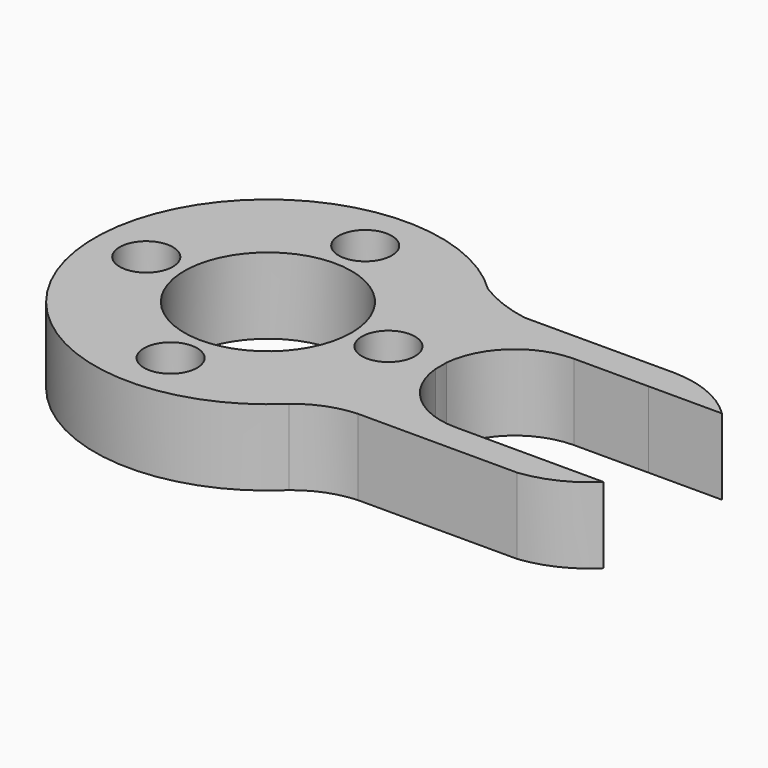
from build123d import *

# Parameters (mm, degrees)
F0_R     = 1.75
F0_R_2   = 5.5
F1_DEPTH = 5


# Not quite as in the source:
# - ends of sketch curves that miss each other by under 0.0002 mm in the source are joined


with BuildPart() as f1:
    # F0 (on Top) → F1 (new body)
    with BuildSketch(Plane.XY):
        with BuildLine():
            ThreePointArc((11.3834703749, 6.8633075193), (9.5916723545, 7.355768815), (7.9272258947, 8.1820110654))
            ThreePointArc((7.9272258947, 8.1820110654), (-11.3923753212, 0), (7.9272258947, -8.1820110654))
            ThreePointArc((7.9272258947, -8.1820110654), (9.5459951376, -7.2276126539), (11.3834703749, -6.8339440851))
            Line((11.3834703749, -6.8339440851), (21.8628461179, -6.8339440851))
            ThreePointArc((21.8628461179, -6.8339440851), (24.0780549828, -6.2025675349), (25.9603803998, -4.874923875))
            Line((25.9603803998, -4.874923875), (21.1398675793, -4.874923875))
            ThreePointArc((21.1398675793, -4.874923875), (21.1127528894, -4.8749999983), (21.0856381954, -4.8749253089))
            ThreePointArc((21.0856381954, -4.8749253089), (21.0855085866, -4.8749245897), (21.0853803998, -4.874923875))
            Line((21.0853803998, -4.874923875), (16.2648675793, -4.874923875))
            ThreePointArc((16.2648675793, -4.874923875), (12.9636398268, -3.6120150473), (11.3834703749, -0.4503528446))
            ThreePointArc((11.3834703749, -0.4503528446), (11.3923753212, 0), (11.3834703749, 0.4503528446))
            ThreePointArc((11.3834703749, 0.4503528446), (12.9535739288, 3.6028655537), (16.2376621588, 4.8749999999))
            Line((16.2376621588, 4.8749999999), (21.1319533126, 4.8749616796))
            Line((21.1319533126, 4.8749616796), (25.9603803998, 4.874923875))
            ThreePointArc((25.9603803998, 4.874923875), (23.8013578283, 6.3274272295), (21.2571545841, 6.8734806254))
            Line((21.2571545841, 6.8734806254), (20.9539298759, 6.8731682053))
            Line((20.9539298759, 6.8731682053), (11.3834703749, 6.8633075193))
        make_face()
        with Locations((0, -8)):
            Circle(F0_R, mode=Mode.SUBTRACT)
        with Locations((-8, 0)):
            Circle(F0_R, mode=Mode.SUBTRACT)
        Circle(F0_R_2, mode=Mode.SUBTRACT)
        with Locations((7.9272258947, 0)):
            Circle(F0_R, mode=Mode.SUBTRACT)
        with Locations((0, 8)):
            Circle(F0_R, mode=Mode.SUBTRACT)
    extrude(amount=F1_DEPTH)


solid = f1.part
